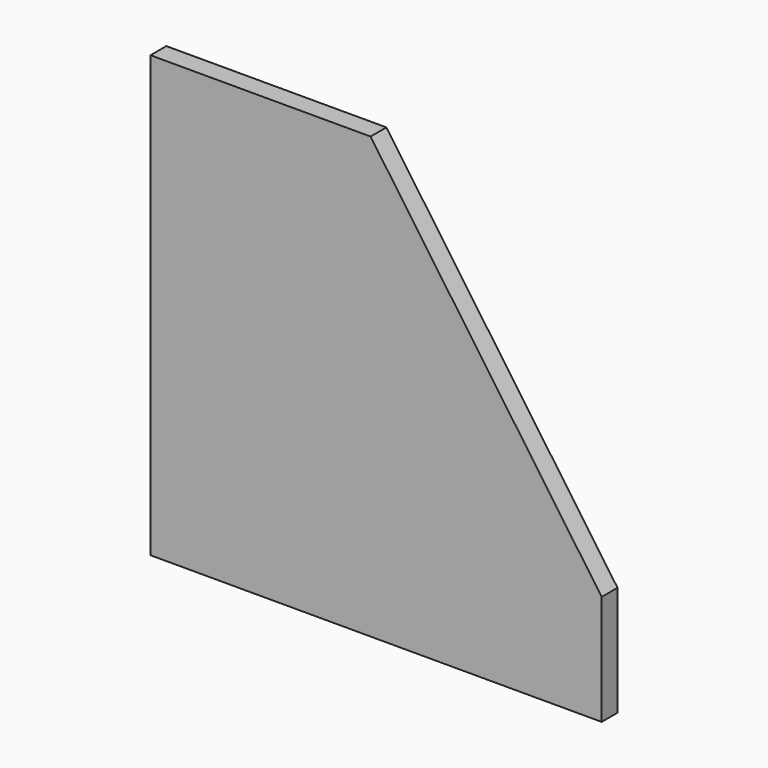
from build123d import *

# Parameters (mm, degrees)
F1_DEPTH = 18


# Not quite as in the source:
# - a feature names something its author has since deleted; it is built from what else it names


with BuildPart() as f1:
    # F0 (on Front) → F1 (new body)
    with BuildSketch(Plane.XZ):
        Polygon((310, -100), (100, 200), (100, -100), align=None)
        Polygon((-100, 200), (-100, -200), (100, -200), (310, -200), (310, -100), (100, -100), (100, 200), align=None)
    extrude(amount=F1_DEPTH)


solid = f1.part
